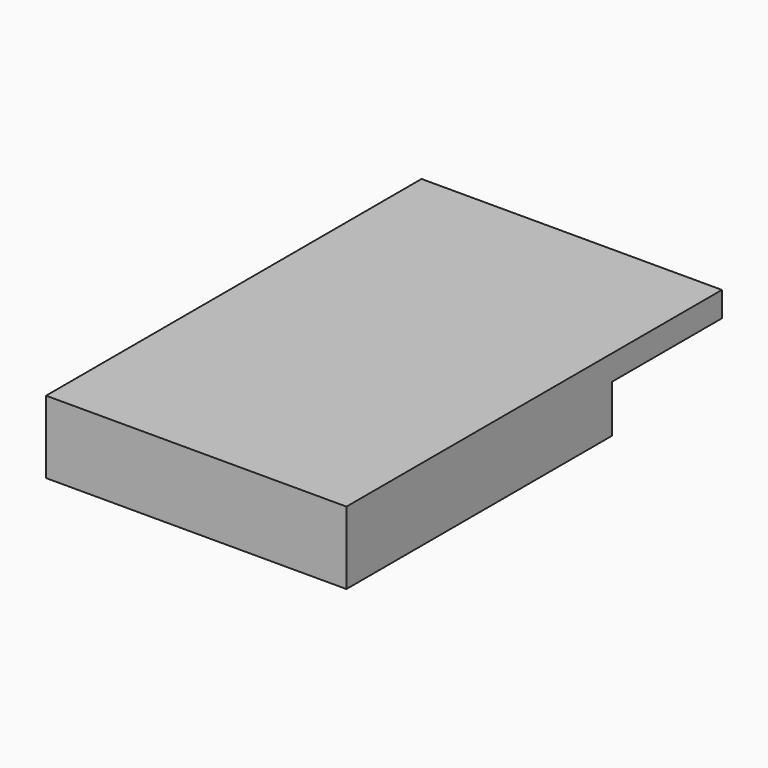
from build123d import *

# Parameters (mm, degrees)
F1_DEPTH = 24.5
F2_W     = 24
F2_H     = 5.8
F3_DEPTH = 2
F4_W     = 24
F4_H     = 11
F4_W_2   = 4.5
F4_H_2   = 2
F5_DEPTH = 2
F6_DEPTH = 1


# Not quite as in the source:
# - a feature of the source that left no trace in its solid (it failed there, or was rolled back) is left out


with BuildPart() as f1:
    # F0 (on Front) → F1 (new body)
    with BuildSketch(Plane.XZ):
        Polygon((-6.75, 2.2), (-6.75, 4.5), (-4.85, 4.5), (-3.2, 4.5), (3.2, 4.5), (4.85, 4.5), (6.75, 4.5), (6.75, 2.2), (4.85, 2.2), (4.85, 0.7), (12.25, 0.7), (12.25, 6.5), (-11.75, 6.5), (-11.75, 0.7), (-4.85, 0.7), (-4.85, 2.2), align=None)
    extrude(amount=F1_DEPTH)

    # F2 (on face) → F3 (join)
    with BuildSketch(Plane.XZ.offset(24.5)):
        with Locations((0.25, 3.6)):
            Rectangle(F2_W, F2_H)
    extrude(amount=F3_DEPTH)

    # F4 (on face) → F5 (join)
    with BuildSketch(Plane.XY.offset(6.5)):
        with Locations((0.25, 5.5)):
            Rectangle(F4_W, F4_H)
        with Locations((0, 7.5)):
            Rectangle(F4_W_2, F4_H_2, mode=Mode.SUBTRACT)
    extrude(amount=-F5_DEPTH)

    # F4 (on face) → F6 (join)
    with BuildSketch(Plane.XY.offset(6.5)):
        with Locations((0, 7.5)):
            Rectangle(F4_W_2, F4_H_2)
    extrude(amount=-F6_DEPTH)


solid = f1.part
